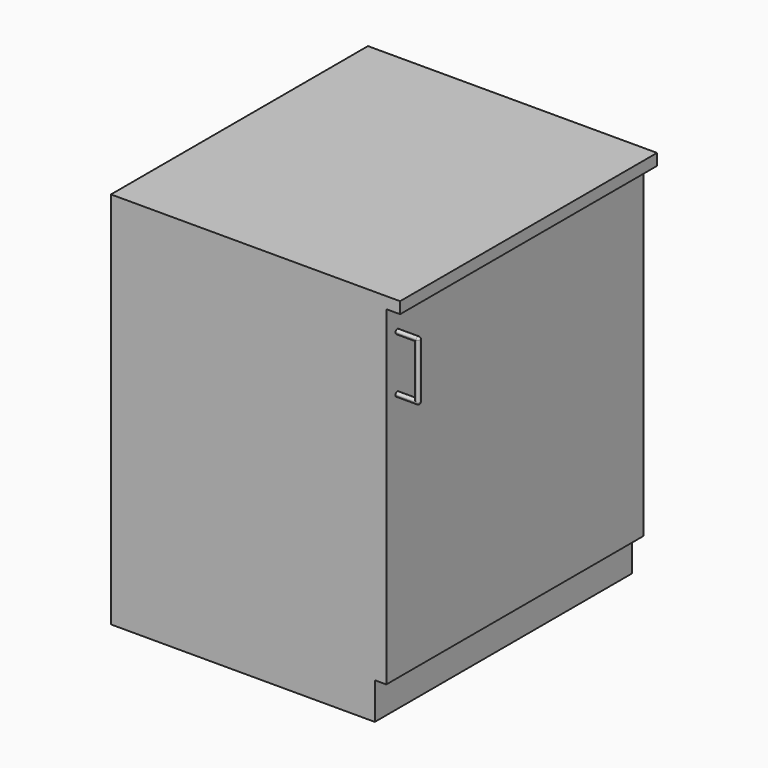
from build123d import *

# Parameters (mm, degrees)
F0_W        = 600
F0_H        = 700
F1_DEPTH    = 800
F2_W        = 700
F2_H        = 80
F3_DEPTH    = 25
F5_DEPTH    = 50
F6_T1_DEPTH = 120
F6_T4_ANGLE = 180
F6_T6_ANGLE = 180
F7_W        = 40
F7_H        = 110
F8_DEPTH    = 25
F9_R        = 4.99999
F10_W       = 630
F10_H       = 700
F11_DEPTH   = 25


# Not quite as in the source:
# - a fillet or chamfer that OpenCascade refuses, or shapes differently, is made with other operations: its cross-section is extruded or revolved along the edge and cut away or added
# - a fillet or chamfer is up to 0.001 mm smaller than in the source, because OpenCascade refuses the exact size


with BuildPart() as f1:
    # F0 (on Top) → F1 (new body)
    with BuildSketch(Plane.XY):
        Rectangle(F0_W, F0_H)
    extrude(amount=F1_DEPTH)

    # F2 (on face) → F3 (cut)
    with BuildSketch(Plane.YZ.offset(300)):
        with Locations((0, 40)):
            Rectangle(F2_W, F2_H)
    extrude(amount=-F3_DEPTH, mode=Mode.SUBTRACT)

    # F4 (on face) → F5 (join)
    with BuildSketch(Plane.YZ.offset(300)):
        with BuildLine():
            ThreePointArc((-320, 750), (-323.5355339059, 748.5355339059), (-325, 745))
            Line((-325, 745), (-325, 625))
            ThreePointArc((-325, 625), (-323.5355339059, 621.4644660941), (-320, 620))
            ThreePointArc((-320, 620), (-316.4644660941, 621.4644660941), (-315, 625))
            Line((-315, 625), (-315, 745))
            ThreePointArc((-315, 745), (-316.4644660941, 748.5355339059), (-320, 750))
        make_face()
    extrude(amount=F5_DEPTH)

    # F6: fillet of radius 5 on 4 edges, made by hand

    # F6_s2 → F6_t1 (cut)
    with BuildSketch(Plane.XY.offset(625)):
        with BuildLine():
            ThreePointArc((345, -325), (348.5355339059, -323.5355339059), (350, -320))
            Line((350, -320), (350, -325))
            Line((350, -325), (345, -325))
        make_face()
        with BuildLine():
            ThreePointArc((345, -315), (348.5355339059, -316.4644660941), (350, -320))
            Line((350, -320), (350, -315))
            Line((350, -315), (345, -315))
        make_face()
    extrude(amount=F6_T1_DEPTH, mode=Mode.SUBTRACT)

    # F6_s3 → F6_t4 (revolve, cut)
    with BuildSketch(Plane.XY.offset(745)):
        with BuildLine():
            ThreePointArc((345, -325), (348.5355339059, -323.5355339059), (350, -320))
            Line((350, -320), (350, -325))
            Line((350, -325), (345, -325))
        make_face()
    revolve(axis=Axis((350, -320, 745), (-1, 0, 0)), revolution_arc=F6_T4_ANGLE, mode=Mode.SUBTRACT)

    # F6_s5 → F6_t6 (revolve, cut)
    with BuildSketch(Plane.XY.offset(625)):
        with BuildLine():
            ThreePointArc((345, -315), (348.5355339059, -316.4644660941), (350, -320))
            Line((350, -320), (350, -315))
            Line((350, -315), (345, -315))
        make_face()
    revolve(axis=Axis((350, -320, 625), (-1, 0, 0)), revolution_arc=F6_T6_ANGLE, mode=Mode.SUBTRACT)

    # F7 (on face) → F8 (cut)
    with BuildSketch(Plane(origin=(0, -315, 0), x_dir=(-1, 0, 0), z_dir=(0, 1, 0))):
        with Locations((-320, 685)):
            Rectangle(F7_W, F7_H)
    extrude(amount=-F8_DEPTH, mode=Mode.SUBTRACT)

    # F9 (radius 5 in the source; OpenCascade refuses exactly that, so slightly less here)
    f9_edges = [f1.edges().sort_by_distance(p)[0] for p in [
        (320, -315, 740),
        (340, -315, 685),
        (320, -315, 630),
        (320, -325, 740),
        (340, -325, 685),
        (320, -325, 630),
    ]]
    fillet(f9_edges, radius=F9_R)

    # F10 (on face) → F11 (join)
    with BuildSketch(Plane.XY.offset(800)):
        with Locations((15, 0)):
            Rectangle(F10_W, F10_H)
    extrude(amount=F11_DEPTH)


solid = f1.part
